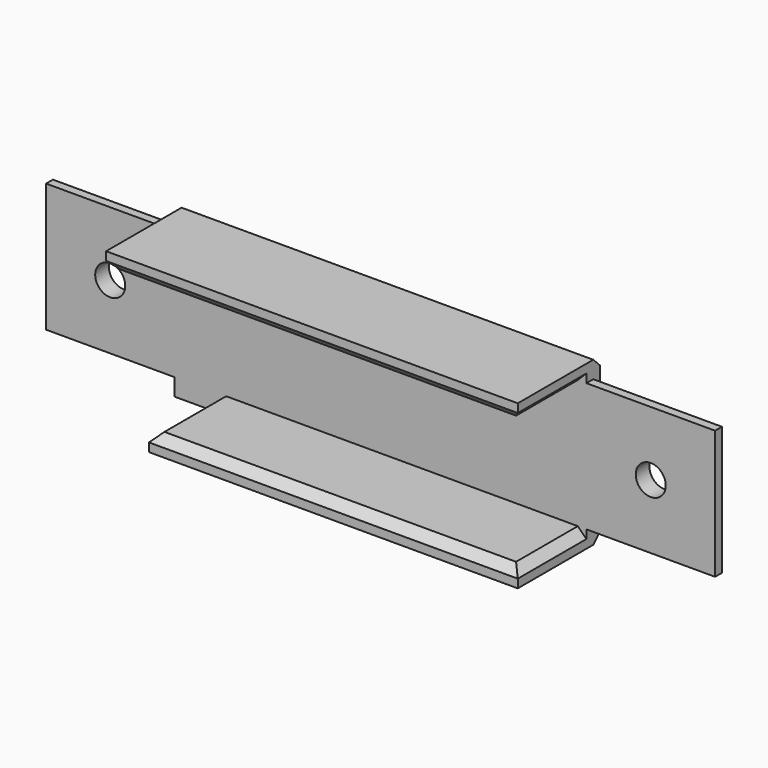
from build123d import *

# Parameters (mm, degrees)
F0_W      = 78
F0_H      = 12
F1_DEPTH  = 19
F2_R      = 1.75
F3_DEPTH  = 10
F3_FACE_W = 15
F3_FACE_H = 2
F2_W      = 15
F2_H      = 2
F4_DEPTH  = 12
F5_SIZE   = 0.99999


# Not quite as in the source:
# - a fillet or chamfer is up to 0.001 mm smaller than in the source, because OpenCascade refuses the exact size


with BuildPart() as f1:
    # F0 (on Top) → F1 (new body)
    with BuildSketch(Plane.XY):
        with Locations((3.4338701516, 6)):
            Rectangle(F0_W, F0_H)
    extrude(amount=-F1_DEPTH)

    # F2 (on face) → F3 (cut)
    with BuildSketch(Plane.XZ):
        Polygon((-35.5661298484, -17), (-20.5661298484, -17), (-20.5661298484, -19), (-15.5661298484, -19), (-15.5661298484, -17), (27.4338701516, -17), (42.4338701516, -17), (42.4338701516, -2), (27.4338701516, -2), (-20.5661298484, -2), (-35.5661298484, -2), align=None)
        with Locations((-28.0890100524, -9.5)):
            Circle(F2_R, mode=Mode.SUBTRACT)
        with Locations((34.9338701516, -9.5)):
            Circle(F2_R, mode=Mode.SUBTRACT)
    extrude(amount=-F3_DEPTH, mode=Mode.SUBTRACT)

    # F3_face (on face) + F2 (on face) → F4 (cut, through all)
    with BuildSketch(Plane(origin=(-28.0661298484, 0, -18), x_dir=(1, 0, 0), z_dir=(0, -1, 0))):
        Rectangle(F3_FACE_W, F3_FACE_H)
    with BuildSketch(Plane.XZ):
        with Locations((-28.0661298484, -1)):
            Rectangle(F2_W, F2_H)
        with Locations((34.9338701516, -1)):
            Rectangle(F2_W, F2_H)
        with Locations((34.9338701516, -18)):
            Rectangle(F2_W, F2_H)
        with Locations((-28.0890100524, -9.5)):
            Circle(F2_R)
        with Locations((34.9338701516, -9.5)):
            Circle(F2_R)
    extrude(amount=-F4_DEPTH, mode=Mode.SUBTRACT)

    # F5 (size 1 in the source; OpenCascade refuses exactly that, so slightly less here)
    f5_edges = [f1.edges().sort_by_distance(p)[0] for p in [
        (-35.56613, 12, -9.5),
        (-28.06613, 12, -2),
        (3.43387, 12, -19),
        (34.93387, 12, -17),
        (42.43387, 12, -9.5),
        (34.93387, 12, -2),
        (3.43387, 12, 0),
        (3.43387, 0, -2),
        (5.93387, 0, -17),
        (27.43387, 5, -17),
        (27.43387, 5, -2),
        (-15.56613, 5, -17),
        (-20.56613, 5, -2),
        (-28.06613, 12, -17),
    ]]
    chamfer(f5_edges, length=F5_SIZE)


solid = f1.part
